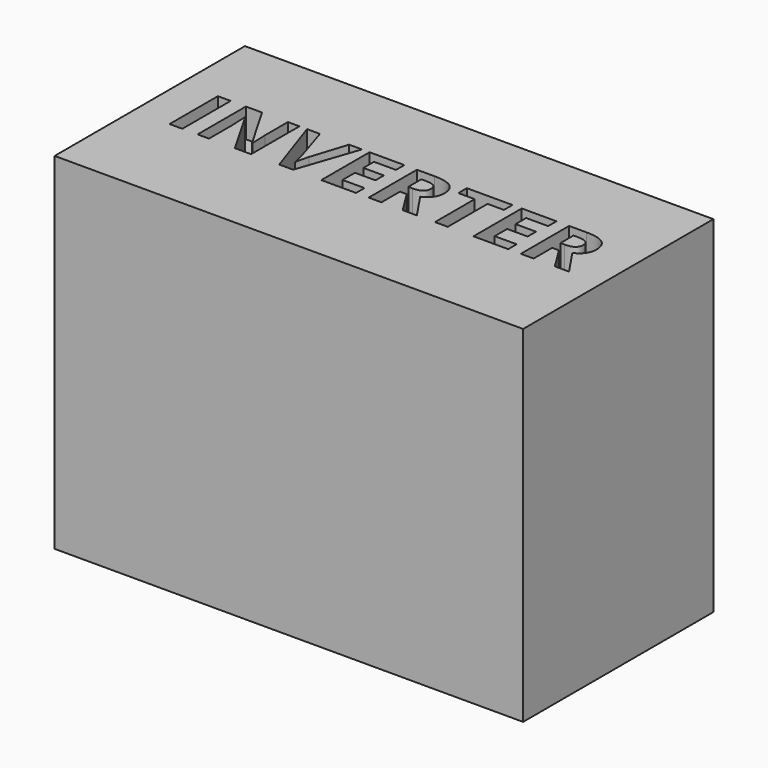
from build123d import *

# Parameters (mm, degrees)
F0_W         = 412.75
F0_H         = 209.55
F1_DEPTH     = 304.8
F2_TEXT_SIZE = 74.5152181647
F3_DEPTH     = 25.4


# Not quite as in the source:
# - Text() gives the source's letters only with a copy of the font that has no kerning and outlines rounded to 1/6400 em; it was checked with that copy


with BuildPart() as f1:
    # F0 (on Top) → F1 (new body)
    with BuildSketch(Plane.XY):
        with Locations((206.375, 104.775)):
            Rectangle(F0_W, F0_H)
    extrude(amount=F1_DEPTH)

    # F2 (on face) → F3 (cut)
    with BuildSketch(Plane.XY.offset(304.8)):
        with Locations((25.4, 86.4517906475)):
            Text('INVERTER', F2_TEXT_SIZE, font='Open Sans', font_style=FontStyle.BOLD, text_align=(TextAlign.LEFT, TextAlign.BOTTOM))
    extrude(amount=-F3_DEPTH, mode=Mode.SUBTRACT)


solid = f1.part
